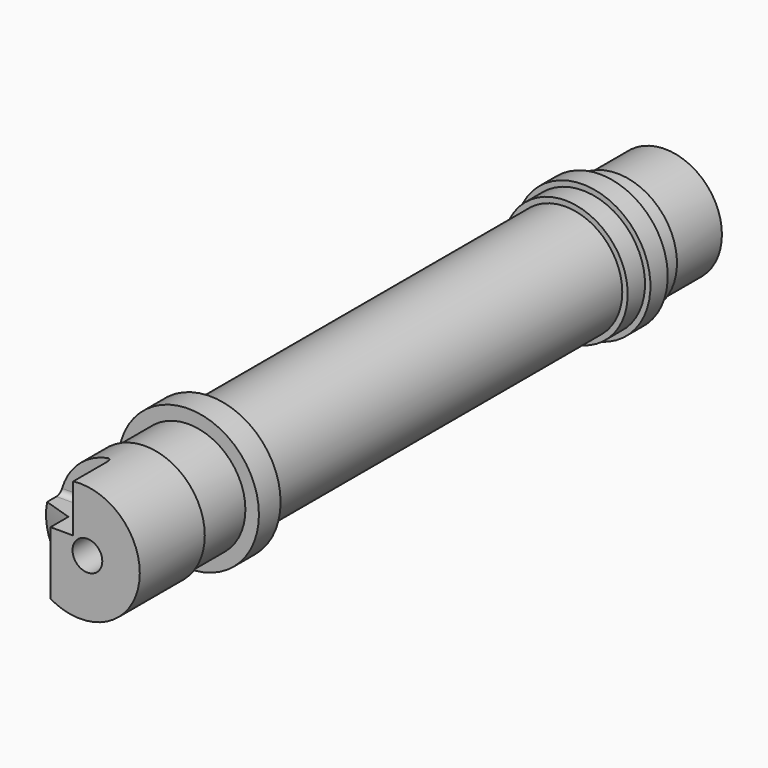
from build123d import *

# Parameters (mm, degrees)
F0_R          = 13
F1_DEPTH      = 5
F2_R          = 10.5
F3_DEPTH      = 25
F3_DEPTH_BACK = 110
F6_START      = -19
F5_R          = 11.5
F5_R_2        = 10.5
F6_DEPTH      = 4
F7_R          = 11
F7_R_2        = 10.5
F8_DEPTH      = 15
F10_DEPTH     = 9
F11_R         = 1
F12_W         = 8.5742305964
F12_H         = 3.8462157547
F13_DEPTH     = 30
F14_T4_ANGLE  = 233.385278584
F16_START     = -15
F15_R         = 12.5
F15_R_2       = 10.5
F16_DEPTH     = 4
F18_START     = -11
F17_R         = 11
F17_R_2       = 10.5
F18_DEPTH     = 3
F19_R         = 2.75
F20_DEPTH     = 148


# Not quite as in the source:
# - a fillet or chamfer that OpenCascade refuses, or shapes differently, is made with other operations: its cross-section is extruded or revolved along the edge and cut away or added


with BuildPart() as f1:
    # F0 (on Front) → F1 (new body)
    with BuildSketch(Plane.XZ):
        Circle(F0_R)
    extrude(amount=F1_DEPTH)

    # F2 (on face) → F3 (join, two sides)
    with BuildSketch(Plane.XZ.offset(5)) as f3_sk:
        Circle(F2_R)
    extrude(amount=F3_DEPTH)
    extrude(f3_sk.sketch, amount=-F3_DEPTH_BACK)

    # F5 (on face) → F6 (join)
    with BuildSketch(Plane(origin=(0, 105, 0), x_dir=(-1, 0, 0), z_dir=(0, 1, 0)).offset(F6_START)):
        Circle(F5_R)
        Circle(F5_R_2, mode=Mode.SUBTRACT)
    extrude(amount=-F6_DEPTH)

    # F7 (on face) → F8 (join)
    with BuildSketch(Plane.XZ.offset(30)):
        Circle(F7_R)
        Circle(F7_R_2, mode=Mode.SUBTRACT)
    extrude(amount=-F8_DEPTH)

    # F9 (on face) → F10 (cut)
    with BuildSketch(Plane.XZ.offset(30)):
        with BuildLine():
            Line((-1.2941175373, 2.1176473238), (-1.2941175373, 10.9243700281))
            ThreePointArc((-1.2941175373, 10.9243700281), (-7.5067341919, 8.0813904617), (-10.8403367922, 2.1176473238))
            Line((-10.8403367922, 2.1176473238), (-1.2941175373, 2.1176473238))
        make_face()
    extrude(amount=-F10_DEPTH, mode=Mode.SUBTRACT)

    # F11
    f11_edges = [f1.edges().sort_by_distance(p)[0] for p in [
        (-6.044178, -21, 2.117647),
        (-1.294118, -21, 6.520629),
    ]]
    fillet(f11_edges, radius=F11_R)

    # F12 (on face) → F13 (cut)
    with BuildSketch(Plane.XY.offset(2.1176473238)):
        with Locations((-9.7801117226, -28.0768921226)):
            Rectangle(F12_W, F12_H)
    extrude(amount=-F13_DEPTH, mode=Mode.SUBTRACT)

    # F14: chamfer of 6 x 2 on 1 edges, made by hand


with BuildPart() as f14_tool2:
    # F14_s3 → F14_t4 (revolve)
    with BuildSketch(Plane(origin=(0, 0, 0), x_dir=(0, 1, 0), z_dir=(0.9992485549, 0, -0.0387598451))):
        Polygon((-24.1537842453, 11), (-26.1537842453, 5), (-26.1537842453, 11), align=None)
    revolve(axis=Axis((0, -26.1537842453, 0), (0, -1, 0)), revolution_arc=F14_T4_ANGLE)

    split(bisect_by=Plane.YZ.offset(-5.4929964244), keep=Keep.BOTTOM)


with BuildPart() as f1_1:
    add(f1.part)

    # F14_t1: cut F14_tool2
    add(f14_tool2.part, mode=Mode.SUBTRACT)

    # F15 (on face) → F16 (join)
    with BuildSketch(Plane(origin=(0, 105, 0), x_dir=(-1, 0, 0), z_dir=(0, 1, 0)).offset(F16_START)):
        Circle(F15_R)
        Circle(F15_R_2, mode=Mode.SUBTRACT)
    extrude(amount=-F16_DEPTH)

    # F17 (on face) → F18 (join)
    with BuildSketch(Plane(origin=(0, 105, 0), x_dir=(-1, 0, 0), z_dir=(0, 1, 0)).offset(F18_START)):
        Circle(F17_R)
        Circle(F17_R_2, mode=Mode.SUBTRACT)
    extrude(amount=-F18_DEPTH)

    # F19 (on face) → F20 (cut)
    with BuildSketch(Plane.XZ.offset(30)):
        with Locations((1.3252417254, -0.3058710963)):
            Circle(F19_R)
    extrude(amount=-F20_DEPTH, mode=Mode.SUBTRACT)


solid = f1_1.part
